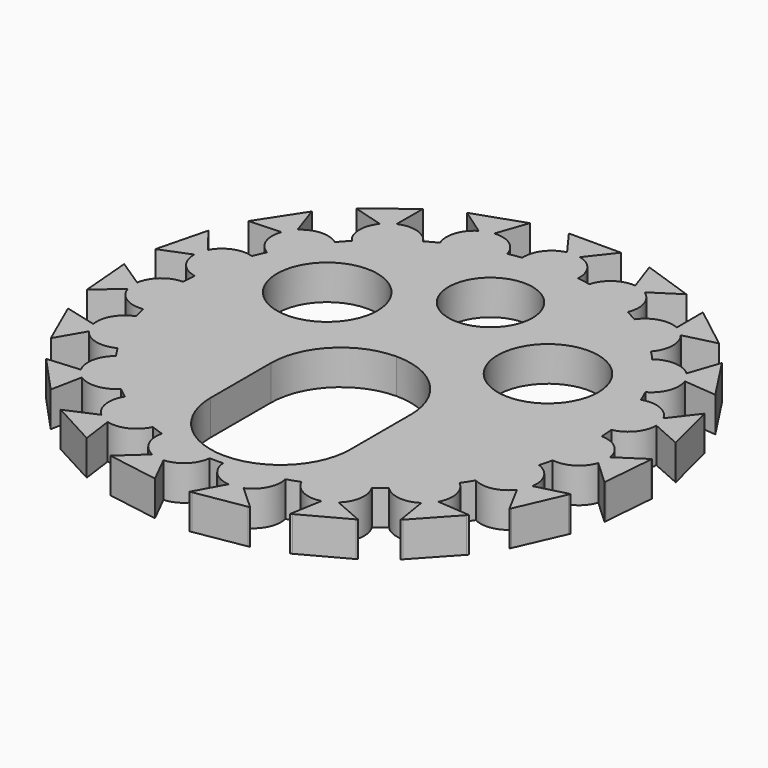
from build123d import *

# Parameters (mm, degrees)
F0_R     = 7.1907441692
F0_R_2   = 6.0113603303
F1_DEPTH = 5


with BuildPart() as f1:
    # F0 (on Top) → F1 (new body)
    with BuildSketch(Plane.XY):
        with BuildLine():
            ThreePointArc((29.3021963996, -6.4328287838), (29.8250389102, -3.235282678), (30, 0))
            ThreePointArc((30, 0), (29.9903388072, 0.7613003555), (29.9613614512, 1.5221103731))
            ThreePointArc((29.9613614512, 1.5221103731), (29.8975347902, 2.4773803642), (29.803258666, 3.4301272408))
            ThreePointArc((29.803258666, 3.4301272408), (29.0820079782, 7.3645646142), (27.8437438152, 11.1680763945))
            ThreePointArc((27.8437438152, 11.1680763945), (27.4731997997, 12.0508627396), (27.0746754108, 12.921375755))
            ThreePointArc((27.0746754108, 12.921375755), (25.1149943479, 16.4084447437), (22.7088244966, 19.603808048))
            ThreePointArc((22.7088244966, 19.603808048), (22.0717173202, 20.3184471488), (21.4121309679, 21.0123927103))
            ThreePointArc((21.4121309679, 21.0123927103), (18.4263813807, 23.6742152819), (15.11305168, 25.9151629151))
            ThreePointArc((15.11305168, 25.9151629151), (14.2784217911, 26.3842125362), (13.4292498912, 26.8263908746))
            ThreePointArc((13.4292498912, 26.8263908746), (9.7409840761, 28.374517251), (5.8795452108, 29.4182077652))
            ThreePointArc((5.8795452108, 29.4182077652), (4.9378377084, 29.5908391021), (3.9911012126, 29.7333333333))
            ThreePointArc((3.9911012126, 29.7333333333), (2, 29.9332590942), (0, 30))
            ThreePointArc((0, 30), (-2, 29.9332590942), (-3.9911012126, 29.7333333333))
            ThreePointArc((-3.9911012126, 29.7333333333), (-4.9378377084, 29.5908391021), (-5.8795452108, 29.4182077652))
            ThreePointArc((-5.8795452108, 29.4182077652), (-9.7409840761, 28.374517251), (-13.4292498912, 26.8263908746))
            ThreePointArc((-13.4292498912, 26.8263908746), (-14.2784217911, 26.3842125362), (-15.11305168, 25.9151629151))
            ThreePointArc((-15.11305168, 25.9151629151), (-18.4263813807, 23.6742152819), (-21.4121309679, 21.0123927103))
            ThreePointArc((-21.4121309679, 21.0123927103), (-22.0717173202, 20.3184471488), (-22.7088244966, 19.603808048))
            ThreePointArc((-22.7088244966, 19.603808048), (-25.1149943479, 16.4084447437), (-27.0746754108, 12.921375755))
            ThreePointArc((-27.0746754108, 12.921375755), (-27.4731997997, 12.0508627396), (-27.8437438152, 11.1680763945))
            ThreePointArc((-27.8437438152, 11.1680763945), (-29.0820079782, 7.3645646142), (-29.803258666, 3.4301272408))
            ThreePointArc((-29.803258666, 3.4301272408), (-29.8975347902, 2.4773803642), (-29.9613614512, 1.5221103731))
            ThreePointArc((-29.9613614512, 1.5221103731), (-29.8975347902, -2.4773803642), (-29.3021963996, -6.4328287838))
            ThreePointArc((-29.3021963996, -6.4328287838), (-29.0820079782, -7.3645646142), (-28.8322006756, -8.2887999252))
            ThreePointArc((-28.8322006756, -8.2887999252), (-27.4731997997, -12.0508627396), (-25.6257864828, -15.5986879941))
            ThreePointArc((-25.6257864828, -15.5986879941), (-25.1149943479, -16.4084447437), (-24.5786235791, -17.2014901377))
            ThreePointArc((-24.5786235791, -17.2014901377), (-22.0717173202, -20.3184471488), (-19.1724249756, -23.0741873217))
            ThreePointArc((-19.1724249756, -23.0741873217), (-18.4263813807, -23.6742152819), (-17.6615712412, -24.2501319851))
            ThreePointArc((-17.6615712412, -24.2501319851), (-14.2784217911, -26.3842125362), (-10.6414337314, -28.04924042))
            ThreePointArc((-10.6414337314, -28.04924042), (-9.7409840761, -28.374517251), (-8.8306136117, -28.6708957523))
            ThreePointArc((-8.8306136117, -28.6708957523), (-4.9378377084, -29.5908391021), (-0.9572780236, -29.98472309))
            ThreePointArc((-0.9572780236, -29.98472309), (0, -30), (0.9572780236, -29.98472309))
            ThreePointArc((0.9572780236, -29.98472309), (4.9378377084, -29.5908391021), (8.8306136117, -28.6708957523))
            ThreePointArc((8.8306136117, -28.6708957523), (9.7409840761, -28.374517251), (10.6414337314, -28.04924042))
            ThreePointArc((10.6414337314, -28.04924042), (14.2784217911, -26.3842125362), (17.6615712412, -24.2501319851))
            ThreePointArc((17.6615712412, -24.2501319851), (18.4263813807, -23.6742152819), (19.1724249756, -23.0741873217))
            ThreePointArc((19.1724249756, -23.0741873217), (22.0717173202, -20.3184471488), (24.5786235791, -17.2014901377))
            ThreePointArc((24.5786235791, -17.2014901377), (25.1149943479, -16.4084447437), (25.6257864828, -15.5986879941))
            ThreePointArc((25.6257864828, -15.5986879941), (27.4731997997, -12.0508627396), (28.8322006756, -8.2887999252))
            ThreePointArc((28.8322006756, -8.2887999252), (29.0820079782, -7.3645646142), (29.3021963996, -6.4328287838))
        make_face()
        with BuildLine():
            Line((-10, -18.4950400144), (-10, -7.7087301761))
            ThreePointArc((-10, -7.7087301761), (-7.0710678119, -0.6376623642), (0, 2.2912698239))
            ThreePointArc((0, 2.2912698239), (7.0710678119, -0.6376623642), (10, -7.7087301761))
            Line((10, -7.7087301761), (10, -18.4950400144))
            ThreePointArc((10, -18.4950400144), (0, -28.4950400144), (-10, -18.4950400144))
        make_face(mode=Mode.SUBTRACT)
        with Locations((-15.8001314849, 9.6030076966)):
            Circle(F0_R, mode=Mode.SUBTRACT)
        with Locations((15.8001314849, 9.6030076966)):
            Circle(F0_R, mode=Mode.SUBTRACT)
        with Locations((0, 19.0711542964)):
            Circle(F0_R_2, mode=Mode.SUBTRACT)
        with BuildLine():
            ThreePointArc((29.9613614512, 1.5221103731), (29.9903388072, 0.7613003555), (30, 0))
            ThreePointArc((30, 0), (29.8250389102, -3.235282678), (29.3021963996, -6.4328287838))
            ThreePointArc((29.3021963996, -6.4328287838), (31.9811449656, -5.8918449835), (33.687382404, -3.7568548909))
            ThreePointArc((33.687382404, -3.7568548909), (33.6967621852, -3.7287281182), (33.7059332236, -3.7005325921))
            ThreePointArc((33.7059332236, -3.7005325921), (33.8838727622, -2.8076977461), (33.8553158726, -1.8977521181))
            ThreePointArc((33.8553158726, -1.8977521181), (33.8509107463, -1.868431639), (33.8462884077, -1.8391446176))
            ThreePointArc((33.8462884077, -1.8391446176), (32.5147296437, 0.5475644451), (29.9613614512, 1.5221103731))
        make_face()
        with BuildLine():
            ThreePointArc((27.8437438152, 11.1680763945), (29.0820079782, 7.3645646142), (29.803258666, 3.4301272408))
            ThreePointArc((29.803258666, 3.4301272408), (32.1613972566, 4.811652224), (33.0819558944, 7.3849770551))
            ThreePointArc((33.0819558944, 7.3849770551), (33.081694705, 7.4146254517), (33.0812137589, 7.4442710977))
            ThreePointArc((33.0812137589, 7.4442710977), (32.9596090419, 8.3465065628), (32.637140581, 9.1978764198))
            ThreePointArc((32.637140581, 9.1978764198), (32.6234537925, 9.2241778923), (32.6095724247, 9.2503771912))
            ThreePointArc((32.6095724247, 9.2503771912), (30.5751980215, 11.0754113497), (27.8437438152, 11.1680763945))
        make_face()
        with BuildLine():
            Line((37.768298191, 0.7490220944), (33.8462884077, -1.8391446176))
            ThreePointArc((33.8462884077, -1.8391446176), (33.8509107463, -1.868431639), (33.8553158726, -1.8977521181))
            Line((33.8553158726, -1.8977521181), (37.7458156921, 0.477698682))
            Line((37.7458156921, 0.477698682), (37.768298191, 0.7490220944))
        make_face()
        with BuildLine():
            ThreePointArc((31.4152338625, -12.7293665698), (30.9307857909, -10.0396195635), (28.8322006756, -8.2887999252))
            ThreePointArc((28.8322006756, -8.2887999252), (27.4731997997, -12.0508627396), (25.6257864828, -15.5986879941))
            ThreePointArc((25.6257864828, -15.5986879941), (28.335239379, -15.9568693657), (30.6422583165, -14.4915733158))
            ThreePointArc((30.6422583165, -14.4915733158), (30.6602626234, -14.4680161392), (30.678091822, -14.4443261558))
            ThreePointArc((30.678091822, -14.4443261558), (31.1362931063, -13.6576444382), (31.4047423701, -12.7877297674))
            ThreePointArc((31.4047423701, -12.7877297674), (31.4100962697, -12.7585676105), (31.4152338625, -12.7293665698))
        make_face()
        with BuildLine():
            ThreePointArc((33.7059332236, -3.7005325921), (33.6967621852, -3.7287281182), (33.687382404, -3.7568548909))
            Line((33.687382404, -3.7568548909), (37.1299028463, -6.9552639756))
            Line((37.1299028463, -6.9552639756), (37.1523853452, -6.6839405632))
            Line((37.1523853452, -6.6839405632), (33.7059332236, -3.7005325921))
        make_face()
        with BuildLine():
            ThreePointArc((33.0812137589, 7.4442710977), (33.081694705, 7.4146254517), (33.0819558944, 7.3849770551))
            Line((33.0819558944, 7.3849770551), (37.3764728157, 5.4776511571))
            Line((37.3764728157, 5.4776511571), (37.3096385829, 5.7415735741))
            Line((37.3096385829, 5.7415735741), (33.0812137589, 7.4442710977))
        make_face()
        with BuildLine():
            Line((37.7458156921, 0.477698682), (33.8553158726, -1.8977521181))
            ThreePointArc((33.8553158726, -1.8977521181), (33.8838727622, -2.8076977461), (33.7059332236, -3.7005325921))
            Line((33.7059332236, -3.7005325921), (37.1523853452, -6.6839405632))
            Line((37.1523853452, -6.6839405632), (37.7458156921, 0.477698682))
        make_face()
        with BuildLine():
            Line((35.9651146952, -11.5549083641), (31.4152338625, -12.7293665698))
            ThreePointArc((31.4152338625, -12.7293665698), (31.4100962697, -12.7585676105), (31.4047423701, -12.7877297674))
            Line((31.4047423701, -12.7877297674), (35.8557517921, -11.8042306702))
            Line((35.8557517921, -11.8042306702), (35.9651146952, -11.5549083641))
        make_face()
        with BuildLine():
            ThreePointArc((22.7088244966, 19.603808048), (25.1149943479, 16.4084447437), (27.0746754108, 12.921375755))
            ThreePointArc((27.0746754108, 12.921375755), (28.8564631193, 14.9937322527), (28.8915861442, 17.7265321475))
            ThreePointArc((28.8915861442, 17.7265321475), (28.8817122881, 17.754489304), (28.8716314755, 17.7823725042))
            ThreePointArc((28.8716314755, 17.7823725042), (28.4636602609, 18.5962373762), (27.88222469, 19.2967723279))
            ThreePointArc((27.88222469, 19.2967723279), (27.8607394153, 19.3172046211), (27.8391032798, 19.337477097))
            ThreePointArc((27.8391032798, 19.337477097), (25.3223692707, 20.4030655819), (22.7088244966, 19.603808048))
        make_face()
        with BuildLine():
            Line((35.4787005423, 12.9717843866), (32.6095724247, 9.2503771912))
            ThreePointArc((32.6095724247, 9.2503771912), (32.6234537925, 9.2241778923), (32.637140581, 9.1978764198))
            Line((32.637140581, 9.1978764198), (35.5455347752, 12.7078619697))
            Line((35.5455347752, 12.7078619697), (35.4787005423, 12.9717843866))
        make_face()
        with BuildLine():
            ThreePointArc((32.637140581, 9.1978764198), (32.9596090419, 8.3465065628), (33.0812137589, 7.4442710977))
            Line((33.0812137589, 7.4442710977), (37.3096385829, 5.7415735741))
            Line((37.3096385829, 5.7415735741), (35.5455347752, 12.7078619697))
            Line((35.5455347752, 12.7078619697), (32.637140581, 9.1978764198))
        make_face()
        with BuildLine():
            ThreePointArc((25.5798512706, -22.2401641377), (25.9950113571, -19.5388550117), (24.5786235791, -17.2014901377))
            ThreePointArc((24.5786235791, -17.2014901377), (22.0717173202, -20.3184471488), (19.1724249756, -23.0741873217))
            ThreePointArc((19.1724249756, -23.0741873217), (21.6187709392, -24.2927193558), (24.2765700768, -23.655904912))
            ThreePointArc((24.2765700768, -23.655904912), (24.3012478635, -23.6394701172), (24.3258031519, -23.6228528538))
            ThreePointArc((24.3258031519, -23.6228528538), (25.0146129629, -23.0275734353), (25.550977737, -22.2919584743))
            ThreePointArc((25.550977737, -22.2919584743), (25.5655104844, -22.2661148118), (25.5798512706, -22.2401641377))
        make_face()
        with BuildLine():
            ThreePointArc((30.678091822, -14.4443261558), (30.6602626234, -14.4680161392), (30.6422583165, -14.4915733158))
            Line((30.6422583165, -14.4915733158), (32.8597317736, -18.6344683345))
            Line((32.8597317736, -18.6344683345), (32.9690946767, -18.3851460285))
            Line((32.9690946767, -18.3851460285), (30.678091822, -14.4443261558))
        make_face()
        with BuildLine():
            Line((35.8557517921, -11.8042306702), (31.4047423701, -12.7877297674))
            ThreePointArc((31.4047423701, -12.7877297674), (31.1362931063, -13.6576444382), (30.678091822, -14.4443261558))
            Line((30.678091822, -14.4443261558), (32.9690946767, -18.3851460285))
            Line((32.9690946767, -18.3851460285), (35.8557517921, -11.8042306702))
        make_face()
        with BuildLine():
            ThreePointArc((28.8716314755, 17.7823725042), (28.8817122881, 17.754489304), (28.8915861442, 17.7265321475))
            Line((28.8915861442, 17.7265321475), (33.5727219999, 17.3169777924))
            Line((33.5727219999, 17.3169777924), (33.4238135614, 17.5448991249))
            Line((33.4238135614, 17.5448991249), (28.8716314755, 17.7823725042))
        make_face()
        with BuildLine():
            Line((30.2645529659, -22.6066852085), (25.5798512706, -22.2401641377))
            ThreePointArc((25.5798512706, -22.2401641377), (25.5655104844, -22.2661148118), (25.550977737, -22.2919584743))
            Line((25.550977737, -22.2919584743), (30.0801608261, -22.8069884677))
            Line((30.0801608261, -22.8069884677), (30.2645529659, -22.6066852085))
        make_face()
        with BuildLine():
            ThreePointArc((15.11305168, 25.9151629151), (18.4263813807, 23.6742152819), (21.4121309679, 21.0123927103))
            ThreePointArc((21.4121309679, 21.0123927103), (22.4244834489, 23.55100874), (21.5703647361, 26.1471424261))
            ThreePointArc((21.5703647361, 26.1471424261), (21.5519481989, 26.170378751), (21.5333599323, 26.193477928))
            ThreePointArc((21.5333599323, 26.193477928), (20.8832322314, 26.8307773195), (20.1058371165, 27.304563534))
            ThreePointArc((20.1058371165, 27.304563534), (20.0788816185, 27.3169124919), (20.0518353264, 27.3290613074))
            ThreePointArc((20.0518353264, 27.3290613074), (17.3254688923, 27.5197310721), (15.11305168, 25.9151629151))
        make_face()
        with BuildLine():
            Line((29.3444351811, 23.7888525627), (27.8391032798, 19.337477097))
            ThreePointArc((27.8391032798, 19.337477097), (27.8607394153, 19.3172046211), (27.88222469, 19.2967723279))
            Line((27.88222469, 19.2967723279), (29.4933436195, 23.5609312302))
            Line((29.4933436195, 23.5609312302), (29.3444351811, 23.7888525627))
        make_face()
        with BuildLine():
            ThreePointArc((27.88222469, 19.2967723279), (28.4636602609, 18.5962373762), (28.8716314755, 17.7823725042))
            Line((28.8716314755, 17.7823725042), (33.4238135614, 17.5448991249))
            Line((33.4238135614, 17.5448991249), (29.4933436195, 23.5609312302))
            Line((29.4933436195, 23.5609312302), (27.88222469, 19.2967723279))
        make_face()
        with BuildLine():
            ThreePointArc((16.9724948814, -29.3408948296), (18.2422740886, -26.9207523428), (17.6615712412, -24.2501319851))
            ThreePointArc((17.6615712412, -24.2501319851), (14.2784217911, -26.3842125362), (10.6414337314, -28.04924042))
            ThreePointArc((10.6414337314, -28.04924042), (12.5595732183, -29.9960762634), (15.2801387795, -30.2567521519))
            ThreePointArc((15.2801387795, -30.2567521519), (15.3088158248, -30.2492207038), (15.3374362566, -30.2414768987))
            ThreePointArc((15.3374362566, -30.2414768987), (16.1822113633, -29.902107541), (16.9283682018, -29.3805075851))
            ThreePointArc((16.9283682018, -29.3805075851), (16.9505049484, -29.360782979), (16.9724948814, -29.3408948296))
        make_face()
        with BuildLine():
            ThreePointArc((24.3258031519, -23.6228528538), (24.3012478635, -23.6394701172), (24.2765700768, -23.655904912))
            Line((24.2765700768, -23.655904912), (25.028698892, -28.2943389058))
            Line((25.028698892, -28.2943389058), (25.2130910318, -28.0940356466))
            Line((25.2130910318, -28.0940356466), (24.3258031519, -23.6228528538))
        make_face()
        with BuildLine():
            Line((30.0801608261, -22.8069884677), (25.550977737, -22.2919584743))
            ThreePointArc((25.550977737, -22.2919584743), (25.0146129629, -23.0275734353), (24.3258031519, -23.6228528538))
            Line((24.3258031519, -23.6228528538), (25.2130910318, -28.0940356466))
            Line((25.2130910318, -28.0940356466), (30.0801608261, -22.8069884677))
        make_face()
        with BuildLine():
            ThreePointArc((21.5333599323, 26.193477928), (21.5519481989, 26.170378751), (21.5703647361, 26.1471424261))
            Line((21.5703647361, 26.1471424261), (26.1308458209, 27.2797411833))
            Line((26.1308458209, 27.2797411833), (25.9159997167, 27.4469626184))
            Line((25.9159997167, 27.4469626184), (21.5333599323, 26.193477928))
        make_face()
        with BuildLine():
            Line((21.2843573199, -31.2086769316), (16.9724948814, -29.3408948296))
            ThreePointArc((16.9724948814, -29.3408948296), (16.9505049484, -29.360782979), (16.9283682018, -29.3805075851))
            Line((16.9283682018, -29.3805075851), (21.0449176929, -31.3382551778))
            Line((21.0449176929, -31.3382551778), (21.2843573199, -31.2086769316))
        make_face()
        with BuildLine():
            ThreePointArc((5.8795452108, 29.4182077652), (9.7409840761, 28.374517251), (13.4292498912, 26.8263908746))
            ThreePointArc((13.4292498912, 26.8263908746), (13.5624630451, 29.5561679988), (11.9116596102, 31.7343041082))
            ThreePointArc((11.9116596102, 31.7343041082), (11.8866961095, 31.7503015851), (11.8616147158, 31.7661135846))
            ThreePointArc((11.8616147158, 31.7661135846), (11.039781953, 32.1577862178), (10.1506701173, 32.3534816072))
            ThreePointArc((10.1506701173, 32.3534816072), (10.1211654424, 32.3564090286), (10.0916398791, 32.3591176711))
            ThreePointArc((10.0916398791, 32.3591176711), (7.4510851272, 31.6542066881), (5.8795452108, 29.4182077652))
        make_face()
        with BuildLine():
            Line((20.0302449421, 32.0280294414), (20.0518353264, 27.3290613074))
            ThreePointArc((20.0518353264, 27.3290613074), (20.0788816185, 27.3169124919), (20.1058371165, 27.304563534))
            Line((20.1058371165, 27.304563534), (20.2450910464, 31.8608080063))
            Line((20.2450910464, 31.8608080063), (20.0302449421, 32.0280294414))
        make_face()
        with BuildLine():
            ThreePointArc((20.1058371165, 27.304563534), (20.8832322314, 26.8307773195), (21.5333599323, 26.193477928))
            Line((21.5333599323, 26.193477928), (25.9159997167, 27.4469626184))
            Line((25.9159997167, 27.4469626184), (20.2450910464, 31.8608080063))
            Line((20.2450910464, 31.8608080063), (20.1058371165, 27.304563534))
        make_face()
        with BuildLine():
            ThreePointArc((6.5259053163, -33.2620842959), (8.5127033645, -31.385368439), (8.8306136117, -28.6708957523))
            ThreePointArc((8.8306136117, -28.6708957523), (4.9378377084, -29.5908391021), (0.9572780236, -29.98472309))
            ThreePointArc((0.9572780236, -29.98472309), (2.1393508573, -32.4488928707), (4.6278673497, -33.5788108142))
            ThreePointArc((4.6278673497, -33.5788108142), (4.6574360507, -33.5809988621), (4.687020158, -33.5829676767))
            ThreePointArc((4.687020158, -33.5829676767), (5.5962160695, -33.5362843157), (6.4713073013, -33.2852228136))
            ThreePointArc((6.4713073013, -33.2852228136), (6.498649187, -33.2737547308), (6.5259053163, -33.2620842959))
        make_face()
        with BuildLine():
            ThreePointArc((15.3374362566, -30.2414768987), (15.3088158248, -30.2492207038), (15.2801387795, -30.2567521519))
            Line((15.2801387795, -30.2567521519), (14.4854181252, -34.8880788248))
            Line((14.4854181252, -34.8880788248), (14.7248577522, -34.7585005786))
            Line((14.7248577522, -34.7585005786), (15.3374362566, -30.2414768987))
        make_face()
        with BuildLine():
            Line((21.0449176929, -31.3382551778), (16.9283682018, -29.3805075851))
            ThreePointArc((16.9283682018, -29.3805075851), (16.1822113633, -29.902107541), (15.3374362566, -30.2414768987))
            Line((15.3374362566, -30.2414768987), (14.7248577522, -34.7585005786))
            Line((14.7248577522, -34.7585005786), (21.0449176929, -31.3382551778))
        make_face()
        with BuildLine():
            ThreePointArc((11.8616147158, 31.7661135846), (11.8866961095, 31.7503015851), (11.9116596102, 31.7343041082))
            Line((11.9116596102, 31.7343041082), (15.8572870353, 34.2863213282))
            Line((15.8572870353, 34.2863213282), (15.5997851744, 34.3747218287))
            Line((15.5997851744, 34.3747218287), (11.8616147158, 31.7661135846))
        make_face()
        with BuildLine():
            Line((9.9976712974, -36.4287242567), (6.5259053163, -33.2620842959))
            ThreePointArc((6.5259053163, -33.2620842959), (6.498649187, -33.2737547308), (6.4713073013, -33.2852228136))
            Line((6.4713073013, -33.2852228136), (9.729131182, -36.4735356764))
            Line((9.729131182, -36.4735356764), (9.9976712974, -36.4287242567))
        make_face()
        with BuildLine():
            ThreePointArc((0, 30), (2, 29.9332590942), (3.9911012126, 29.7333333333))
            ThreePointArc((3.9911012126, 29.7333333333), (3.2307393271, 32.3584578437), (0.9621413371, 33.8825615317))
            ThreePointArc((0.9621413371, 33.8825615317), (0.9333360554, 33.8895865857), (0.904479493, 33.8963979323))
            ThreePointArc((0.904479493, 33.8963979323), (0.4551968096, 33.9740150811), (0, 34))
            Line((0, 34), (0, 30))
        make_face()
        with BuildLine():
            Line((8.5454668624, 36.7964723642), (10.0916398791, 32.3591176711))
            ThreePointArc((10.0916398791, 32.3591176711), (10.1211654424, 32.3564090286), (10.1506701173, 32.3534816072))
            Line((10.1506701173, 32.3534816072), (8.8029687233, 36.7080718637))
            Line((8.8029687233, 36.7080718637), (8.5454668624, 36.7964723642))
        make_face()
        with BuildLine():
            ThreePointArc((10.1506701173, 32.3534816072), (11.039781953, 32.1577862178), (11.8616147158, 31.7661135846))
            Line((11.8616147158, 31.7661135846), (15.5997851744, 34.3747218287))
            Line((15.5997851744, 34.3747218287), (8.8029687233, 36.7080718637))
            Line((8.8029687233, 36.7080718637), (10.1506701173, 32.3534816072))
        make_face()
        with BuildLine():
            ThreePointArc((-4.687020158, -33.5829676767), (-2.160612591, -32.4695576793), (-0.9572780236, -29.98472309))
            ThreePointArc((-0.9572780236, -29.98472309), (-4.9378377084, -29.5908391021), (-8.8306136117, -28.6708957523))
            ThreePointArc((-8.8306136117, -28.6708957523), (-8.5127033645, -31.385368439), (-6.5259053163, -33.2620842959))
            ThreePointArc((-6.5259053163, -33.2620842959), (-5.6254429477, -33.5312958059), (-4.687020158, -33.5829676767))
        make_face()
        with BuildLine():
            ThreePointArc((4.687020158, -33.5829676767), (4.6574360507, -33.5809988621), (4.6278673497, -33.5788108142))
            Line((4.6278673497, -33.5788108142), (2.3724175401, -37.7011540587))
            Line((2.3724175401, -37.7011540587), (2.6409576554, -37.6563426391))
            Line((2.6409576554, -37.6563426391), (4.687020158, -33.5829676767))
        make_face()
        with BuildLine():
            Line((9.729131182, -36.4735356764), (6.4713073013, -33.2852228136))
            ThreePointArc((6.4713073013, -33.2852228136), (5.5962160695, -33.5362843157), (4.687020158, -33.5829676767))
            Line((4.687020158, -33.5829676767), (2.6409576554, -37.6563426391))
            Line((2.6409576554, -37.6563426391), (9.729131182, -36.4735356764))
        make_face()
        with BuildLine():
            ThreePointArc((-3.9911012126, 29.7333333333), (-2, 29.9332590942), (0, 30))
            Line((0, 30), (0, 34))
            ThreePointArc((0, 34), (-0.4551968096, 33.9740150811), (-0.904479493, 33.8963979323))
            ThreePointArc((-0.904479493, 33.8963979323), (-3.2131688914, 32.3823403777), (-3.9911012126, 29.7333333333))
        make_face()
        with BuildLine():
            ThreePointArc((0.904479493, 33.8963979323), (0.9333360554, 33.8895865857), (0.9621413371, 33.8825615317))
            Line((0.9621413371, 33.8825615317), (3.8653451484, 37.5774465501))
            Line((3.8653451484, 37.5774465501), (3.593091853, 37.5774465501))
            Line((3.593091853, 37.5774465501), (0.904479493, 33.8963979323))
        make_face()
        with BuildLine():
            Line((-2.6409576554, -37.6563426391), (-4.687020158, -33.5829676767))
            ThreePointArc((-4.687020158, -33.5829676767), (-5.6254429477, -33.5312958059), (-6.5259053163, -33.2620842959))
            Line((-6.5259053163, -33.2620842959), (-9.9976712974, -36.4287242567))
            Line((-9.9976712974, -36.4287242567), (-2.6409576554, -37.6563426391))
        make_face()
        with BuildLine():
            ThreePointArc((-0.904479493, 33.8963979323), (-0.4551968096, 33.9740150811), (0, 34))
            ThreePointArc((0, 34), (0.4551968096, 33.9740150811), (0.904479493, 33.8963979323))
            Line((0.904479493, 33.8963979323), (3.593091853, 37.5774465501))
            Line((3.593091853, 37.5774465501), (-3.593091853, 37.5774465501))
            Line((-3.593091853, 37.5774465501), (-0.904479493, 33.8963979323))
        make_face()
        with BuildLine():
            ThreePointArc((-15.3374362566, -30.2414768987), (-12.586392785, -30.0087177221), (-10.6414337314, -28.04924042))
            ThreePointArc((-10.6414337314, -28.04924042), (-14.2784217911, -26.3842125362), (-17.6615712412, -24.2501319851))
            ThreePointArc((-17.6615712412, -24.2501319851), (-18.2422740886, -26.9207523428), (-16.9724948814, -29.3408948296))
            ThreePointArc((-16.9724948814, -29.3408948296), (-16.2082348821, -29.8878993707), (-15.3374362566, -30.2414768987))
        make_face()
        with BuildLine():
            ThreePointArc((-13.4292498912, 26.8263908746), (-9.7409840761, 28.374517251), (-5.8795452108, 29.4182077652))
            ThreePointArc((-5.8795452108, 29.4182077652), (-7.4510851272, 31.6542066881), (-10.0916398791, 32.3591176711))
            ThreePointArc((-10.0916398791, 32.3591176711), (-11.0117034126, 32.1673094109), (-11.8616147158, 31.7661135846))
            ThreePointArc((-11.8616147158, 31.7661135846), (-13.5535992703, 29.5844616223), (-13.4292498912, 26.8263908746))
        make_face()
        with BuildLine():
            Line((-14.7248577522, -34.7585005786), (-15.3374362566, -30.2414768987))
            ThreePointArc((-15.3374362566, -30.2414768987), (-16.2082348821, -29.8878993707), (-16.9724948814, -29.3408948296))
            Line((-16.9724948814, -29.3408948296), (-21.2843573199, -31.2086769316))
            Line((-21.2843573199, -31.2086769316), (-14.7248577522, -34.7585005786))
        make_face()
        with BuildLine():
            ThreePointArc((-11.8616147158, 31.7661135846), (-11.0117034126, 32.1673094109), (-10.0916398791, 32.3591176711))
            Line((-10.0916398791, 32.3591176711), (-8.5454668624, 36.7964723642))
            Line((-8.5454668624, 36.7964723642), (-15.5997851744, 34.3747218287))
            Line((-15.5997851744, 34.3747218287), (-11.8616147158, 31.7661135846))
        make_face()
        with BuildLine():
            ThreePointArc((-24.3258031519, -23.6228528538), (-21.6482420227, -24.2959675664), (-19.1724249756, -23.0741873217))
            ThreePointArc((-19.1724249756, -23.0741873217), (-22.0717173202, -20.3184471488), (-24.5786235791, -17.2014901377))
            ThreePointArc((-24.5786235791, -17.2014901377), (-25.9950113571, -19.5388550117), (-25.5798512706, -22.2401641377))
            ThreePointArc((-25.5798512706, -22.2401641377), (-25.0346130703, -23.00568528), (-24.3258031519, -23.6228528538))
        make_face()
        with BuildLine():
            ThreePointArc((-21.4121309679, 21.0123927103), (-18.4263813807, 23.6742152819), (-15.11305168, 25.9151629151))
            ThreePointArc((-15.11305168, 25.9151629151), (-17.3254688923, 27.5197310721), (-20.0518353264, 27.3290613074))
            ThreePointArc((-20.0518353264, 27.3290613074), (-20.8597672396, 26.8489016068), (-21.5333599323, 26.193477928))
            ThreePointArc((-21.5333599323, 26.193477928), (-22.4252868624, 23.5806473999), (-21.4121309679, 21.0123927103))
        make_face()
        with BuildLine():
            Line((-25.2130910318, -28.0940356466), (-24.3258031519, -23.6228528538))
            ThreePointArc((-24.3258031519, -23.6228528538), (-25.0346130703, -23.00568528), (-25.5798512706, -22.2401641377))
            Line((-25.5798512706, -22.2401641377), (-30.2645529659, -22.6066852085))
            Line((-30.2645529659, -22.6066852085), (-25.2130910318, -28.0940356466))
        make_face()
        with BuildLine():
            ThreePointArc((-21.5333599323, 26.193477928), (-20.8597672396, 26.8489016068), (-20.0518353264, 27.3290613074))
            Line((-20.0518353264, 27.3290613074), (-20.0302449421, 32.0280294414))
            Line((-20.0302449421, 32.0280294414), (-25.9159997167, 27.4469626184))
            Line((-25.9159997167, 27.4469626184), (-21.5333599323, 26.193477928))
        make_face()
        with BuildLine():
            ThreePointArc((-30.678091822, -14.4443261558), (-28.3641683302, -15.9503723341), (-25.6257864828, -15.5986879941))
            ThreePointArc((-25.6257864828, -15.5986879941), (-27.4731997997, -12.0508627396), (-28.8322006756, -8.2887999252))
            ThreePointArc((-28.8322006756, -8.2887999252), (-30.9307857909, -10.0396195635), (-31.4152338625, -12.7293665698))
            ThreePointArc((-31.4152338625, -12.7293665698), (-31.1481024803, -13.6304482193), (-30.678091822, -14.4443261558))
        make_face()
        with BuildLine():
            ThreePointArc((-27.0746754108, 12.921375755), (-25.1149943479, 16.4084447437), (-22.7088244966, 19.603808048))
            ThreePointArc((-22.7088244966, 19.603808048), (-25.3223692707, 20.4030655819), (-27.8391032798, 19.337477097))
            ThreePointArc((-27.8391032798, 19.337477097), (-28.4473516135, 18.6209987101), (-28.8716314755, 17.7823725042))
            ThreePointArc((-28.8716314755, 17.7823725042), (-28.8668466588, 15.0215041403), (-27.0746754108, 12.921375755))
        make_face()
        with BuildLine():
            Line((-32.9690946767, -18.3851460285), (-30.678091822, -14.4443261558))
            ThreePointArc((-30.678091822, -14.4443261558), (-31.1481024803, -13.6304482193), (-31.4152338625, -12.7293665698))
            Line((-31.4152338625, -12.7293665698), (-35.9651146952, -11.5549083641))
            Line((-35.9651146952, -11.5549083641), (-32.9690946767, -18.3851460285))
        make_face()
        with BuildLine():
            ThreePointArc((-28.8716314755, 17.7823725042), (-28.4473516135, 18.6209987101), (-27.8391032798, 19.337477097))
            Line((-27.8391032798, 19.337477097), (-29.3444351811, 23.7888525627))
            Line((-29.3444351811, 23.7888525627), (-33.4238135614, 17.5448991249))
            Line((-33.4238135614, 17.5448991249), (-28.8716314755, 17.7823725042))
        make_face()
        with BuildLine():
            ThreePointArc((-33.7059332236, -3.7005325921), (-32.0063968837, -5.8763067639), (-29.3021963996, -6.4328287838))
            ThreePointArc((-29.3021963996, -6.4328287838), (-29.8975347902, -2.4773803642), (-29.9613614512, 1.5221103731))
            ThreePointArc((-29.9613614512, 1.5221103731), (-32.5147296437, 0.5475644451), (-33.8462884077, -1.8391446176))
            ThreePointArc((-33.8462884077, -1.8391446176), (-33.886211674, -2.7781405959), (-33.7059332236, -3.7005325921))
        make_face()
        with BuildLine():
            ThreePointArc((-29.803258666, 3.4301272408), (-29.0820079782, 7.3645646142), (-27.8437438152, 11.1680763945))
            ThreePointArc((-27.8437438152, 11.1680763945), (-30.5751980215, 11.0754113497), (-32.6095724247, 9.2503771912))
            ThreePointArc((-32.6095724247, 9.2503771912), (-32.952224034, 8.3752216685), (-33.0812137589, 7.4442710977))
            ThreePointArc((-33.0812137589, 7.4442710977), (-32.1802357044, 4.8345478245), (-29.803258666, 3.4301272408))
        make_face()
        with BuildLine():
            Line((-37.1523853452, -6.6839405632), (-33.7059332236, -3.7005325921))
            ThreePointArc((-33.7059332236, -3.7005325921), (-33.886211674, -2.7781405959), (-33.8462884077, -1.8391446176))
            Line((-33.8462884077, -1.8391446176), (-37.768298191, 0.7490220944))
            Line((-37.768298191, 0.7490220944), (-37.1523853452, -6.6839405632))
        make_face()
        with BuildLine():
            ThreePointArc((-33.0812137589, 7.4442710977), (-32.952224034, 8.3752216685), (-32.6095724247, 9.2503771912))
            Line((-32.6095724247, 9.2503771912), (-35.4787005423, 12.9717843866))
            Line((-35.4787005423, 12.9717843866), (-37.3096385829, 5.7415735741))
            Line((-37.3096385829, 5.7415735741), (-33.0812137589, 7.4442710977))
        make_face()
    extrude(amount=F1_DEPTH)


solid = f1.part
